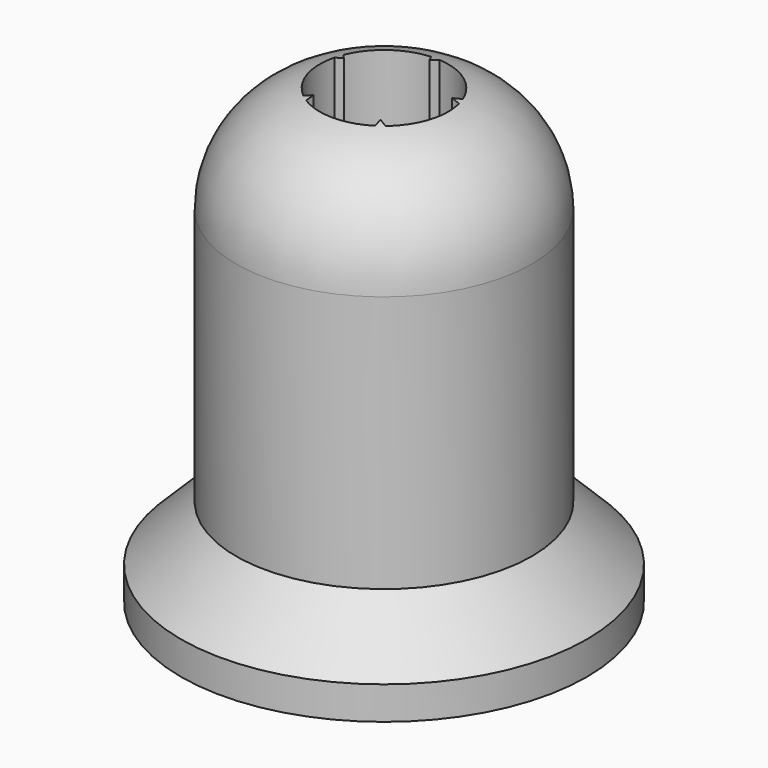
from build123d import *

# Parameters (mm, degrees)
F0_R     = 11.05
F0_R_2   = 2.6
F1_DEPTH = 1.8
F2_R     = 11.05
F2_R_2   = 2.6
F3_DEPTH = 3
F4_SIZE  = 2.99999
F5_R     = 8.05
F6_DEPTH = 20


# Not quite as in the source:
# - a fillet or chamfer that OpenCascade refuses, or shapes differently, is made with other operations: its cross-section is extruded or revolved along the edge and cut away or added
# - a fillet or chamfer is up to 0.001 mm smaller than in the source, because OpenCascade refuses the exact size


with BuildPart() as f1:
    # F0 (on Top) → F1 (new body)
    with BuildSketch(Plane.XY):
        Circle(F0_R)
        Circle(F0_R_2, mode=Mode.SUBTRACT)
    extrude(amount=F1_DEPTH)


with BuildPart() as f3:
    # F2 (on face) → F3 (new body)
    with BuildSketch(Plane.XY.offset(1.8)):
        Circle(F2_R)
        Circle(F2_R_2, mode=Mode.SUBTRACT)
    extrude(amount=F3_DEPTH)

    # F4 (size 3 in the source; OpenCascade refuses exactly that, so slightly less here)
    f4_edges = [f3.edges().sort_by_distance(p)[0] for p in [
        (-11.05, 0, 4.8),
    ]]
    chamfer(f4_edges, length=F4_SIZE)

    # F5 (on face) → F6 (join)
    with BuildSketch(Plane.XY.offset(4.8)):
        Circle(F5_R)
        with BuildLine():
            ThreePointArc((-3.2516549392, 1.2948900171), (-2.057248383, 2.8315594803), (-0.2266969526, 3.4926506398))
            Line((-0.2266969526, 3.4926506398), (0, 3.1))
            Line((0, 3.1), (0.2266969526, 3.4926506398))
            ThreePointArc((0.2266969526, 3.4926506398), (2.057248383, 2.8315594803), (3.2516549392, 1.2948900171))
            Line((3.2516549392, 1.2948900171), (2.9482752005, 0.9579526826))
            Line((2.9482752005, 0.9579526826), (3.391761361, 0.8636867891))
            ThreePointArc((3.391761361, 0.8636867891), (3.328697807, -1.0815594803), (2.2363302247, -2.6923645975))
            Line((2.2363302247, -2.6923645975), (1.8221342821, -2.5079526826))
            Line((1.8221342821, -2.5079526826), (1.8695268503, -2.9588628485))
            ThreePointArc((1.8695268503, -2.9588628485), (0, -3.5), (-1.8695268503, -2.9588628485))
            Line((-1.8695268503, -2.9588628485), (-1.8221342821, -2.5079526826))
            Line((-1.8221342821, -2.5079526826), (-2.2363302247, -2.6923645975))
            ThreePointArc((-2.2363302247, -2.6923645975), (-3.328697807, -1.0815594803), (-3.391761361, 0.8636867891))
            Line((-3.391761361, 0.8636867891), (-2.9482752005, 0.9579526826))
            Line((-2.9482752005, 0.9579526826), (-3.2516549392, 1.2948900171))
        make_face(mode=Mode.SUBTRACT)
    extrude(amount=F6_DEPTH)

    # F7: fillet of radius 6 on 1 edges, made by hand

    # F7_s1 → F7_t2 (revolve, cut)
    with BuildSketch(Plane.XZ):
        with BuildLine():
            ThreePointArc((8.05, 18.8), (6.2926406871, 23.0426406871), (2.05, 24.8))
            Line((2.05, 24.8), (8.05, 24.8))
            Line((8.05, 24.8), (8.05, 18.8))
        make_face()
    revolve(axis=Axis((0, 0, 24.8), (0, 0, 1)), mode=Mode.SUBTRACT)


solid = Compound([f1.part, f3.part])
